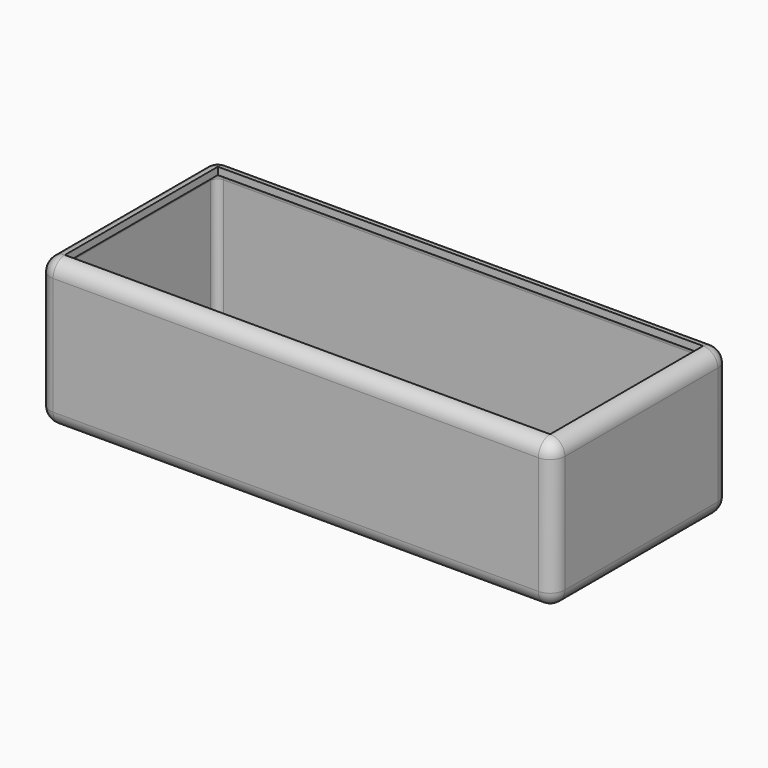
from build123d import *

# Parameters (mm, degrees)
F0_W     = 177.8
F0_H     = 50.8
F1_DEPTH = 76.2
F2_R     = 5.08
F3_T     = -2.54


# Not quite as in the source:
# - a shell that OpenCascade refuses in one call is made with other operations: the cavity is built on its own and cut out


with BuildPart() as f1:
    # F0 (on Front) → F1 (new body)
    with BuildSketch(Plane.XZ):
        with Locations((88.9, 25.4)):
            Rectangle(F0_W, F0_H)
    extrude(amount=F1_DEPTH)

    # F2
    f2_edges = [f1.edges().sort_by_distance(p)[0] for p in [
        (88.9, -76.2, 50.8),
        (177.8, -38.1, 50.8),
        (177.8, -76.2, 25.4),
        (88.9, -76.2, 0),
        (177.8, -38.1, 0),
        (177.8, 0, 25.4),
        (88.9, 0, 50.8),
        (0, 0, 25.4),
        (88.9, 0, 0),
        (0, -38.1, 50.8),
        (0, -38.1, 0),
        (0, -76.2, 25.4),
    ]]
    fillet(f2_edges, radius=F2_R)

    # F3: a shell. OpenCascade refuses it in one call, so the cavity is built on its own and cut out:
    # the body offset inwards by the wall thickness, plus a prism from it out through each open face.
    f3_core = offset(f1.part, amount=F3_T, mode=Mode.PRIVATE)
    f3_exits = [f3_core.faces().sort_by_distance(p)[0] for p in [
        (88.9, -38.1, 48.26),
    ]]
    add(f3_core, mode=Mode.SUBTRACT)
    extrude(f3_exits, amount=-F3_T, mode=Mode.SUBTRACT)


solid = f1.part
